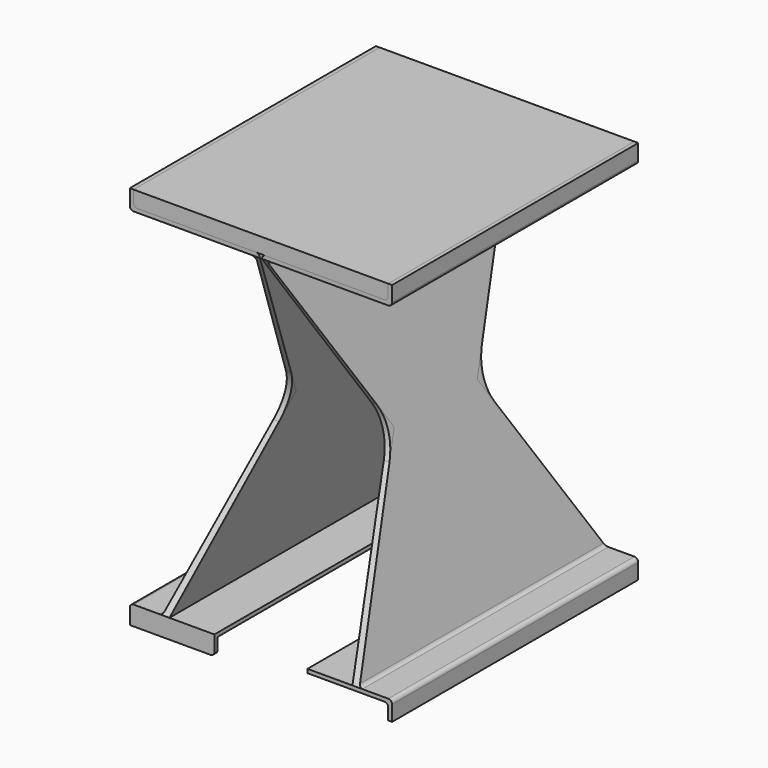
from build123d import *

# Parameters (mm, degrees)
F2_DEPTH     = 400
F4_DEPTH     = 784
F5_R         = 5
F6_T4_DEPTH  = 183.8018686822
F6_T10_DEPTH = 183.8018686822
F9_DEPTH     = 5
F11_DEPTH    = 5
F13_W        = 331
F13_H        = 5
F14_DEPTH    = 390
F16_DEPTH    = 5
F18_DEPTH    = 5


# Not quite as in the source:
# - a fillet or chamfer that OpenCascade refuses, or shapes differently, is made with other operations: its cross-section is extruded or revolved along the edge and cut away or added


with BuildPart() as f2:
    # F1 (on Front) → F2 (new body)
    with BuildSketch(Plane.XZ):
        Polygon((-118.9635416667, -475), (0, -20), (-165.5, -20), (-165.5, 0), (-170.5, 0), (-170.5, -25), (-6.4646408415, -25), (-128.0534928563, -475), (-170.5, -475), (-170.5, -500), (-165.5, -500), (-165.5, -480), (-60.5, -480), (-60.5, -475), align=None)
    extrude(amount=F2_DEPTH)

    # F3 (on Right) → F4 (cut)
    with BuildSketch(Plane.YZ):
        Polygon((162.0724052191, -25), (0, -25), (-132.508663875, -250), (0, -475), (162.0724052191, -475), align=None)
        Polygon((-267.491336125, -250), (-400, -25), (-562.0724052191, -25), (-562.0724052191, -475), (-400, -475), align=None)
    extrude(amount=-F4_DEPTH, mode=Mode.SUBTRACT)

    # F5
    f5_edges = [f2.edges().sort_by_distance(p)[0] for p in [
        (-6.464641, -200, -25),
        (0, -200, -20),
        (-170.5, -200, -25),
        (-165.5, -200, -20),
        (-128.053493, -200, -475),
        (-170.5, -200, -475),
        (-165.5, -200, -480),
    ]]
    fillet(f5_edges, radius=F5_R)

    # F6: fillet of radius 60 on 2 edges, made by hand


with BuildPart() as f6_tool2:
    # F6_s3 → F6_t4 (new body)
    with BuildSketch(Plane.YZ.offset(28.2036925833)):
        with BuildLine():
            ThreePointArc((-114.5771279689, -219.5522129582), (-122.8767192253, -250), (-114.5771279689, -280.4477870418))
            Line((-114.5771279689, -280.4477870418), (-132.508663875, -250))
            Line((-132.508663875, -250), (-114.5771279689, -219.5522129582))
        make_face()
    extrude(amount=-F6_T4_DEPTH)

    split(bisect_by=Plane(origin=(4.8945715066, 0, -1.2797265085), x_dir=(0, 1, 0), z_dir=(-0.9674779969, 0, 0.2529551846)), keep=Keep.TOP)

    split(bisect_by=Plane(origin=(0.2705438763, 0, -0.0731002652), x_dir=(0, 1, 0), z_dir=(0.9653810975, 0, -0.2608435098)), keep=Keep.TOP)


with BuildPart() as f2_1:
    add(f2.part)

    # F6_t1: union F6_tool2
    add(f6_tool2.part)


with BuildPart() as f6_tool8:
    # F6_s9 → F6_t10 (new body)
    with BuildSketch(Plane.YZ.offset(28.2036925833)):
        with BuildLine():
            ThreePointArc((-285.4228720311, -219.5522129582), (-277.1232807747, -250), (-285.4228720311, -280.4477870418))
            Line((-285.4228720311, -280.4477870418), (-267.491336125, -250))
            Line((-267.491336125, -250), (-285.4228720311, -219.5522129582))
        make_face()
    extrude(amount=-F6_T10_DEPTH)

    split(bisect_by=Plane(origin=(4.8945715066, 0, -1.2797265085), x_dir=(0, 1, 0), z_dir=(-0.9674779969, 0, 0.2529551846)), keep=Keep.TOP)

    split(bisect_by=Plane(origin=(0.2705438763, 0, -0.0731002652), x_dir=(0, 1, 0), z_dir=(0.9653810975, 0, -0.2608435098)), keep=Keep.TOP)


with BuildPart() as f2_2:
    add(f2_1.part)

    # F6_t7: union F6_tool8
    add(f6_tool8.part)


with BuildPart() as f7_1:
    # F7: instance of F2
    add(f2_2.part.mirror(Plane.YZ))


with BuildPart() as f9:
    # F8 (on Front) → F9 (new body)
    with BuildSketch(Plane.XZ):
        with BuildLine():
            Line((165.5, 0), (-165.5, 0))
            Line((-165.5, 0), (-165.5, -15))
            ThreePointArc((-165.5, -15), (-164.0355339059, -18.5355339059), (-160.5, -20))
            Line((-160.5, -20), (-6.4753678563, -20))
            Line((-6.4753678563, -20), (160.5, -20))
            ThreePointArc((160.5, -20), (164.0355339059, -18.5355339059), (165.5, -15))
            Line((165.5, -15), (165.5, 0))
        make_face()
    extrude(amount=F9_DEPTH)



with BuildPart() as f11:
    # F10 (on face) → F11 (new body)
    with BuildSketch(Plane.XZ.offset(400)):
        with BuildLine():
            Line((165.5, 0), (-165.5, 0))
            Line((-165.5, 0), (-165.5, -15))
            ThreePointArc((-165.5, -15), (-164.0355339059, -18.5355339059), (-160.5, -20))
            Line((-160.5, -20), (-6.4753678563, -20))
            Line((-6.4753678563, -20), (160.5, -20))
            ThreePointArc((160.5, -20), (164.0355339059, -18.5355339059), (165.5, -15))
            Line((165.5, -15), (165.5, 0))
        make_face()
    extrude(amount=-F11_DEPTH)


with BuildPart() as f9_1:
    add(f9.part)

    add(f11.part)  # F14 merges F11
    # F13 (on face) → F14 (join, through all)
    with BuildSketch(Plane(origin=(0, -395, 0), x_dir=(-1, 0, 0), z_dir=(0, 1, 0))):
        with Locations((0, -2.5)):
            Rectangle(F13_W, F13_H)
    extrude(amount=F14_DEPTH)


with BuildPart() as f16:
    # F15 (on face) → F16 (new body)
    with BuildSketch(Plane(origin=(0, 0, 0), x_dir=(-1, 0, 0), z_dir=(0, 1, 0))):
        with BuildLine():
            ThreePointArc((165.5, -485), (164.0355339059, -481.4644660941), (160.5, -480))
            Line((160.5, -480), (60.5, -480))
            Line((60.5, -480), (60.5, -495))
            ThreePointArc((60.5, -495), (61.9644660941, -498.5355339059), (65.5, -500))
            Line((65.5, -500), (165.5, -500))
            Line((165.5, -500), (165.5, -485))
        make_face()
    extrude(amount=-F16_DEPTH)


with BuildPart() as f2_3:
    add(f2_2.part)

    # F17 (on face) → F18 (join)
    with BuildSketch(Plane.XZ.offset(400)):
        with BuildLine():
            ThreePointArc((-160.5, -480), (-164.0355339059, -481.4644660941), (-165.5, -485))
            Line((-165.5, -485), (-165.5, -500))
            Line((-165.5, -500), (-65.5, -500))
            ThreePointArc((-65.5, -500), (-61.9644660941, -498.5355339059), (-60.5, -495))
            Line((-60.5, -495), (-60.5, -480))
            Line((-60.5, -480), (-160.5, -480))
        make_face()
    extrude(amount=-F18_DEPTH)


solid = Compound([f7_1.part, f9_1.part, f16.part, f2_3.part])
